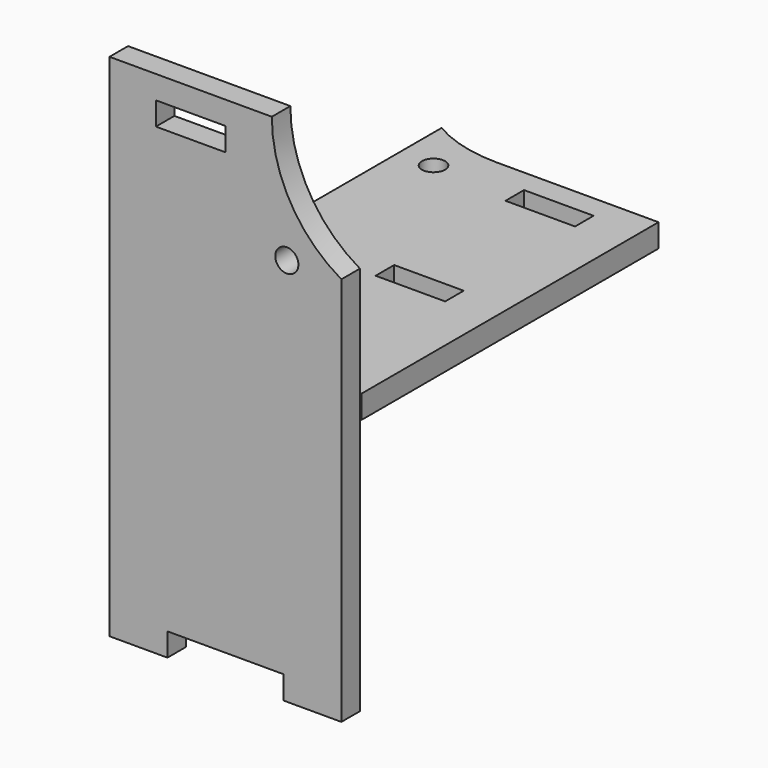
from build123d import *

# Parameters (mm, degrees)
F0_W     = 30
F0_H     = 10
F0_R     = 5
F1_DEPTH = 10
F2_W     = 30
F2_H     = 10
F2_R     = 5
F3_DEPTH = 10


# Not quite as in the source:
# - a feature names something its author has since deleted; it is built from what else it names


with BuildPart() as f1:
    # F0 (on Front) → F1 (new body)
    with BuildSketch(Plane.XZ):
        with BuildLine():
            ThreePointArc((50, 58.0384757729), (28.0384757729, 80), (20, 110))
            Line((20, 110), (-50, 110))
            Line((-50, 110), (-50, -110))
            Line((-50, -110), (-25, -110))
            Line((-25, -110), (-25, -100))
            Line((-25, -100), (25, -100))
            Line((25, -100), (25, -110))
            Line((25, -110), (50, -110))
            Line((50, -110), (50, 58.0384757729))
        make_face()
        with Locations((-15, 95)):
            Rectangle(F0_W, F0_H, mode=Mode.SUBTRACT)
        with Locations((26.4736674726, 57.5719177723)):
            Circle(F0_R, mode=Mode.SUBTRACT)
    extrude(amount=F1_DEPTH)


with BuildPart() as f3:
    # F2 (on Top) → F3 (new body)
    with BuildSketch(Plane.XY):
        with BuildLine():
            ThreePointArc((-20.2736711096, 161.2976664366), (-35.8028138157, 163.3421168592), (-50.2736711096, 169.3361422095))
            Line((-50.2736711096, 169.3361422095), (-50.2736711096, 1.2976664366))
            Line((-50.2736711096, 1.2976664366), (-25.2736711096, 1.2976664366))
            Line((-25.2736711096, 1.2976664366), (-25.2736711096, 11.2976664366))
            Line((-25.2736711096, 11.2976664366), (24.7263288904, 11.2976664366))
            Line((24.7263288904, 11.2976664366), (24.7263288904, 1.2976664366))
            Line((24.7263288904, 1.2976664366), (49.7263288904, 1.2976664366))
            Line((49.7263288904, 1.2976664366), (49.7263288904, 161.2976664366))
            Line((49.7263288904, 161.2976664366), (-20.2736711096, 161.2976664366))
        make_face()
        with Locations((14.7263288904, 76.2976664366)):
            Rectangle(F2_W, F2_H, mode=Mode.SUBTRACT)
        with Locations((-35.3022602503, 146.2976664366)):
            Circle(F2_R, mode=Mode.SUBTRACT)
        with Locations((14.7263288904, 146.2976664366)):
            Rectangle(F2_W, F2_H, mode=Mode.SUBTRACT)
    extrude(amount=F3_DEPTH)


solid = Compound([f1.part, f3.part])
